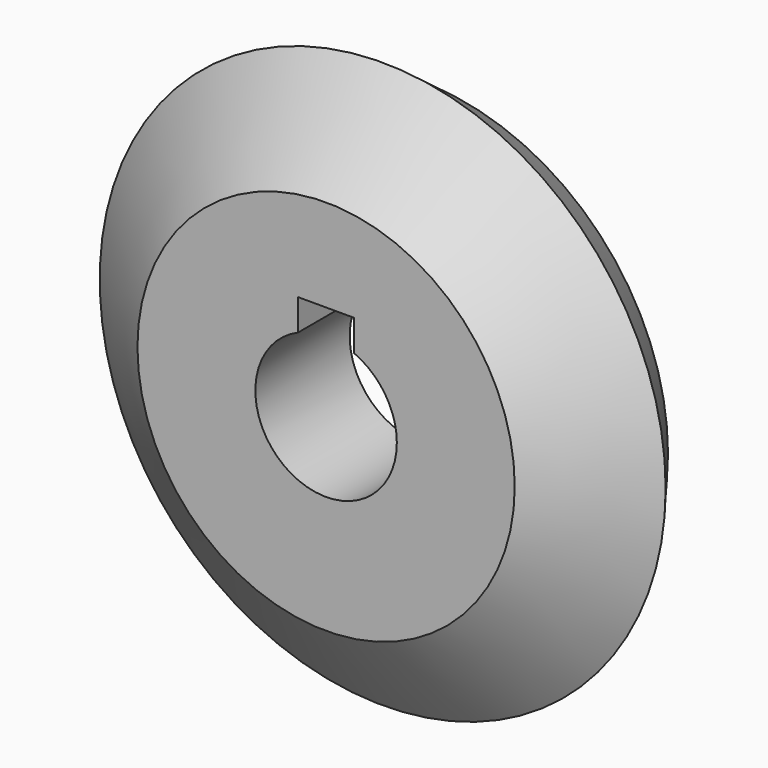
from build123d import *

# Parameters (mm, degrees)
F0_R     = 60
F1_DEPTH = 25
F2_SIZE2 = 7.5
F2_SIZE  = 10
F3_SIZE2 = 14.99999
F3_SIZE  = 19.99999


# Not quite as in the source:
# - a fillet or chamfer is up to 0.001 mm smaller than in the source, because OpenCascade refuses the exact size


with BuildPart() as f1:
    # F0 (on Front) → F1 (new body)
    with BuildSketch(Plane.XZ):
        Circle(F0_R)
        with BuildLine():
            ThreePointArc((5.9278272092, 13.7790008556), (12.5283160907, 8.2487148048), (15, 0))
            ThreePointArc((15, 0), (-8.2487148048, -12.5283160907), (-5.9278272092, 13.7790008556))
            Line((-5.9278272092, 13.7790008556), (-5.9278272092, 20.3793700784))
            Line((-5.9278272092, 20.3793700784), (5.9278272092, 20.3793700784))
            Line((5.9278272092, 20.3793700784), (5.9278272092, 13.7790008556))
        make_face(mode=Mode.SUBTRACT)
    extrude(amount=F1_DEPTH)

    # F2
    f2_edges = [f1.edges().sort_by_distance(p)[0] for p in [
        (-60, 0, 0),
    ]]
    f2_side = f1.faces().sort_by_distance((-60, -12.5, 0))[0]
    chamfer(f2_edges, length=F2_SIZE, length2=F2_SIZE2, reference=f2_side)

    # F3 (size 20 and 15 in the source; OpenCascade refuses exactly that, so slightly less here)
    f3_edges = [f1.edges().sort_by_distance(p)[0] for p in [
        (-60, -25, 0),
    ]]
    f3_side = f1.faces().sort_by_distance((-58.302944, -25, 0))[0]
    chamfer(f3_edges, length=F3_SIZE, length2=F3_SIZE2, reference=f3_side)


solid = f1.part
